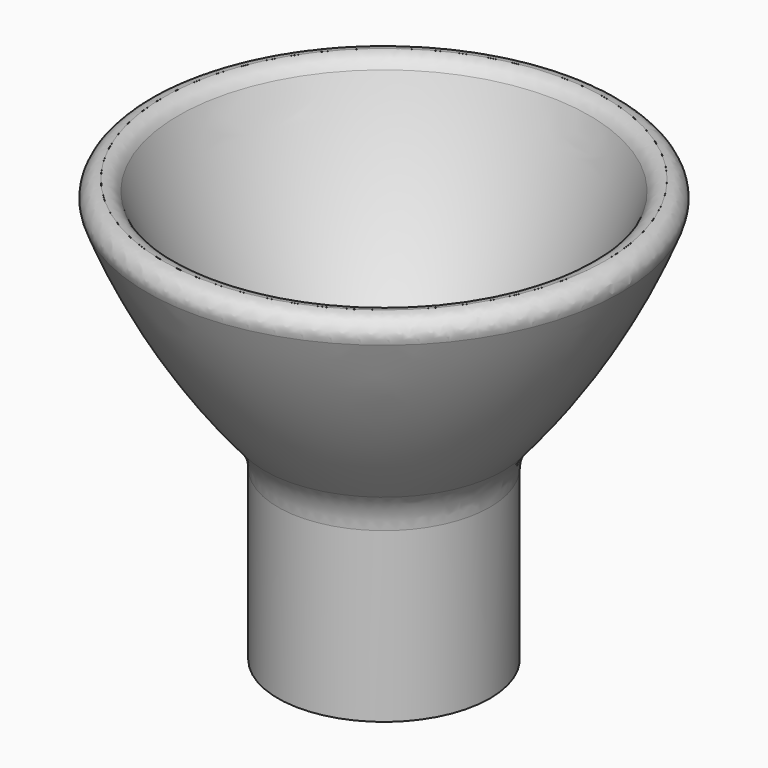
from build123d import *

# Parameters (mm, degrees)
F2_W     = 70.9480602289
F2_H     = 11.2090441923
F3_DEPTH = 25
F4_R     = 1.4999
F5_R     = 5


# Not quite as in the source:
# - a fillet or chamfer is up to 0.001 mm smaller than in the source, because OpenCascade refuses the exact size


with BuildPart() as f1:
    # F0 (on Front) → F1 (revolve)
    with BuildSketch(Plane.XZ):
        with BuildLine():
            Line((6.48, 15), (6.48, 0))
            Line((6.48, 0), (9.48, 0))
            Line((9.48, 0), (9.48, 16.9443072909))
            ThreePointArc((9.48, 16.9443072909), (18.4709094822, 29.8049687465), (23.8669980317, 44.5398014486))
            Line((23.8669980317, 44.5398014486), (23.8669980317, 44.6510324618))
            ThreePointArc((23.8669980317, 44.6510324618), (23.4276582035, 45.7116926336), (22.3669980317, 46.1510324618))
            Line((22.3669980317, 46.1510324618), (22.3540474458, 46.1510324618))
            ThreePointArc((22.3540474458, 46.1510324618), (21.4193322825, 45.8241938162), (20.8919518365, 44.9861092131))
            ThreePointArc((20.8919518365, 44.9861092131), (15.376267951, 30.3745650676), (6.1462926992, 17.7758529155))
            Line((6.1462926992, 17.7758529155), (6.1462926992, 17.4685423841))
            Line((6.1462926992, 17.4685423841), (6.1462926992, 15.7758529155))
            ThreePointArc((6.1462926992, 15.7758529155), (5.9998460898, 15.4222995249), (5.6462926992, 15.2758529155))
            Line((5.6462926992, 15.2758529155), (4.9462926992, 15.2758529155))
            Line((4.9462926992, 15.2758529155), (4.9462926992, 14.7758529155))
            Line((4.9462926992, 14.7758529155), (6.48, 15))
        make_face()
    revolve(axis=Axis((0, 0, 18.4), (0, 0, 1)))

    # F2 (on Front) → F3 (cut, symmetric)
    with BuildSketch(Plane.XZ):
        with Locations((3.8653966039, 43.3803750116)):
            Rectangle(F2_W, F2_H)
    extrude(amount=F3_DEPTH, both=True, mode=Mode.SUBTRACT)

    # F4 (radius 1.5 in the source; OpenCascade refuses exactly that, so slightly less here)
    f4_edges = [f1.edges().sort_by_distance(p)[0] for p in [
        (-21.925894, 0, 37.775853),
        (-18.736377, 0, 37.775853),
    ]]
    fillet(f4_edges, radius=F4_R)

    # F5
    f5_edges = [f1.edges().sort_by_distance(p)[0] for p in [
        (-9.48, 0, 16.944307),
    ]]
    fillet(f5_edges, radius=F5_R)


solid = f1.part
